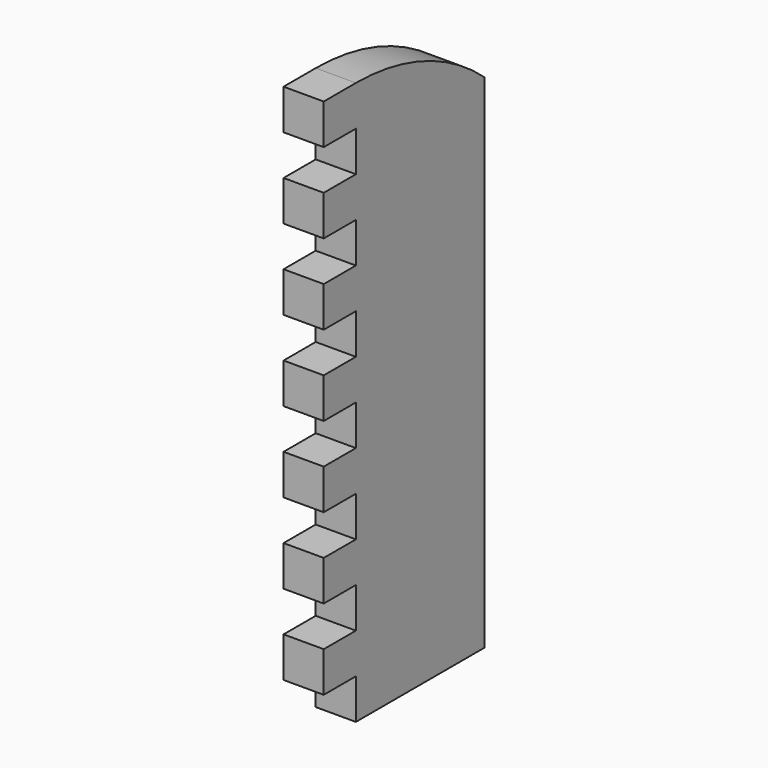
from build123d import *

# Parameters (mm, degrees)
F0_W     = 100
F0_H     = 280
F1_DEPTH = 20
F3_DEPTH = 20
F4_W     = 20
F4_H     = 20
F5_DEPTH = 20


# Not quite as in the source:
# - a feature names something its author has since deleted; it is built from what else it names


with BuildPart() as f1:
    # F0 (on Right) → F1 (new body)
    with BuildSketch(Plane.YZ):
        Rectangle(F0_W, F0_H)
    extrude(amount=F1_DEPTH)

    # F2 (on face) → F3 (cut, through all)
    with BuildSketch(Plane.YZ.offset(20)):
        with BuildLine():
            ThreePointArc((-30, 140), (12.7200187266, 132.2533832709), (50, 110))
            Line((50, 110), (50, 140))
            Line((50, 140), (-30, 140))
        make_face()
    extrude(amount=-F3_DEPTH, mode=Mode.SUBTRACT)

    # F4 (on face) → F5 (cut, through all)
    with BuildSketch(Plane(origin=(0, 0, 0), x_dir=(0, -1, 0), z_dir=(-1, 0, 0))):
        with Locations((40, -130)):
            Rectangle(F4_W, F4_H)
        with Locations((40, -90)):
            Rectangle(F4_W, F4_H)
        with Locations((40, -50)):
            Rectangle(F4_W, F4_H)
        with Locations((40, -10)):
            Rectangle(F4_W, F4_H)
        with Locations((40, 30)):
            Rectangle(F4_W, F4_H)
        with Locations((40, 70)):
            Rectangle(F4_W, F4_H)
        with Locations((40, 110)):
            Rectangle(F4_W, F4_H)
    extrude(amount=-F5_DEPTH, mode=Mode.SUBTRACT)


solid = f1.part
